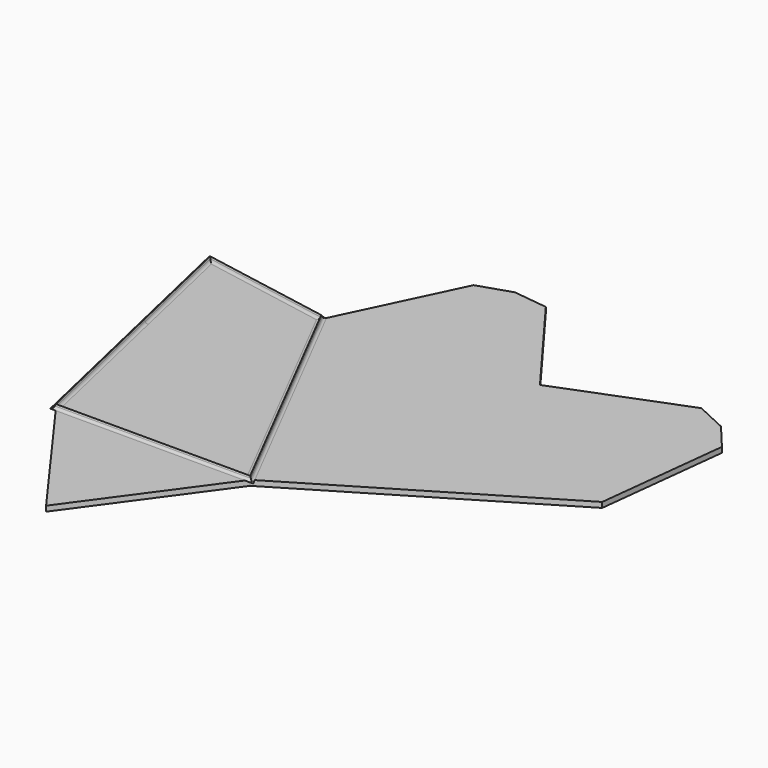
from build123d import *

# Parameters (mm, degrees)
F1_DEPTH = 3


# Not quite as in the source:
# - a feature names something its author has since deleted; it is built from what else it names


with BuildPart() as f1:
    # F0 (on Top) → F1 (new body)
    with BuildSketch(Plane.XY):
        Polygon((-28.4502197635, 72.6983953348), (-51.6819700906, -29.8425633773), (-23.1152368132, 17.8982210566), align=None)
        Polygon((-140.7768225768, -22.2294077159), (-10.6683637709, -109.9542610041), (-51.6819700906, -29.8425633773), align=None)
        Polygon((-51.6819700906, -29.8425633773), (-10.6683637709, -109.9542610041), (-23.1152368132, 17.8982210566), align=None)
        Polygon((-10.6683637709, -109.9542610041), (-120.6683637709, -109.9542610041), (-65.6683637709, -185.6552666301), align=None)
        Polygon((132.4114346114, 44.946839524), (66.5490740882, -63.721509729), (124.0331667167, -29.3037948908), align=None)
        Polygon((-140.7768225768, -22.2294077159), (-120.6683637709, -109.9542610041), (-10.6683637709, -109.9542610041), align=None)
        Polygon((-155.7464530213, 43.0768719543), (-140.7768225768, -22.2294077159), (-51.6819700906, -29.8425633773), align=None)
        Polygon((-155.7464530213, 43.0768719543), (-51.6819700906, -29.8425633773), (-82.214321462, 29.796144856), align=None)
        Polygon((-82.214321462, 29.796144856), (-51.6819700906, -29.8425633773), (-49.9971651586, 97.2157779285), align=None)
        Polygon((67.6016469638, -8.0965797169), (-10.6683637709, -109.9542610041), (66.5490740882, -63.721509729), align=None)
        Polygon((-31.4300453332, 103.3067331799), (-49.9971651586, 97.2157779285), (-28.4502197635, 72.6983953348), align=None)
        Polygon((-31.4300453332, 103.3067331799), (-28.4502197635, 72.6983953348), (-12.0367519986, 100.9113529511), align=None)
        Polygon((-12.0367519508, 100.9113529867), (14.1232700197, -23.4361999186), (32.5792640638, 40.9716900005), align=None)
        Polygon((119.8878838282, 59.9467845327), (101.1497655445, 35.5616942262), (132.4114345522, 44.9468395307), align=None)
        Polygon((102.1690833879, 68.1858247536), (101.1497655445, 35.5616942262), (119.8878838282, 59.9467845327), align=None)
        Polygon((32.5792640638, 40.9716900005), (14.1232700197, -23.4361999186), (102.1690833662, 68.185824809), align=None)
        Polygon((-49.9971651586, 97.2157779285), (-51.6819700906, -29.8425633773), (-28.4502197635, 72.6983953348), align=None)
        Polygon((-28.4502197635, 72.6983953348), (-23.1152368132, 17.8982210566), (14.1232700197, -23.4361999186), align=None)
        Polygon((-23.1152368132, 17.8982210566), (-10.6683637709, -109.9542610041), (14.1232700197, -23.4361999186), align=None)
        Polygon((-28.4502197635, 72.6983953348), (14.1232700197, -23.4361999186), (-12.0367519508, 100.9113529867), align=None)
        Polygon((14.1232700197, -23.4361999186), (-10.6683637709, -109.9542610041), (67.6016469638, -8.0965797169), align=None)
        Polygon((102.1690833662, 68.185824809), (14.1232700197, -23.4361999186), (101.1497655445, 35.5616942262), align=None)
        Polygon((101.1497655445, 35.5616942262), (66.5490740882, -63.721509729), (132.4114346114, 44.946839524), align=None)
        Polygon((67.6016469638, -8.0965797169), (66.5490740882, -63.721509729), (101.1497655445, 35.5616942262), align=None)
        Polygon((101.1497655445, 35.5616942262), (14.1232700197, -23.4361999186), (67.6016469638, -8.0965797169), align=None)
    extrude(amount=F1_DEPTH)

    # F6: sweep along a path in F2
    with BuildLine(Plane.XY.offset(3)) as f6_path:
        Line((-10.6683637709, -109.9542610041), (-51.6819700906, -29.8425633773))
        Line((-51.6819700906, -29.8425633773), (-82.214321462, 29.796144856))
        Line((-82.214321462, 29.796144856), (-155.7464530213, 43.0768719543))
        Line((-155.7464530213, 43.0768719543), (-140.7768225768, -22.2294077159))
        Line((-140.7768225768, -22.2294077159), (-120.6683637709, -109.9542610041))
        Line((-120.6683637709, -109.9542610041), (-10.6683637709, -109.9542610041))
    # F5 (on plane+point) → F6 (sweep)
    with BuildSketch(Plane.YZ.offset(-120.6683637709)):
        with BuildLine():
            Line((-111.9542610041, 3), (-107.9542610041, 3))
            add(Edge.make_bspline(
                [(-107.9542610041, 3), (-108.6989912072, 3), (-109.1337455213, 3.0200950451), (-109.5714134942, 4.0761884477)],
                knots=[0, 0, 0, 0, 1.9425148007, 1.9425148007, 1.9425148007, 1.9425148007], degree=3))
            Line((-109.5714134942, 4.0761884477), (-109.9542610041, 5))
            Line((-109.9542610041, 5), (-110.3371085141, 4.0761884477))
            add(Edge.make_bspline(
                [(-111.9542610041, 3), (-111.2095308011, 3), (-110.774776487, 3.0200950451), (-110.3371085141, 4.0761884477)],
                knots=[0, 0, 0, 0, 1.9425148007, 1.9425148007, 1.9425148007, 1.9425148007], degree=3))
        make_face()
    sweep(path=f6_path.line, transition=Transition.RIGHT)


solid = f1.part
